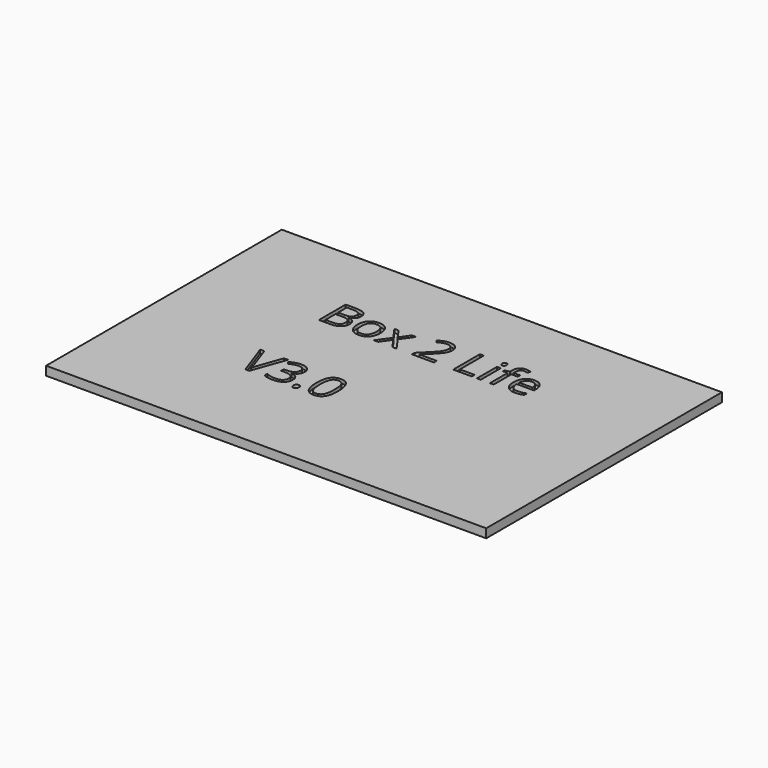
from build123d import *

# Parameters (mm, degrees)
F0_W         = 124
F0_H         = 83
F1_DEPTH     = 2.5
F2_TEXT_SIZE = 13.1944444444
F3_DEPTH     = 1


# Not quite as in the source:
# - Text() gives the source's letters only with a copy of the font that has no kerning and outlines rounded to 1/6400 em; it was checked with that copy


with BuildPart() as f1:
    # F0 (on Top) → F1 (new body)
    with BuildSketch(Plane.XY):
        with Locations((62, 41.5)):
            Rectangle(F0_W, F0_H)
    extrude(amount=F1_DEPTH)

    # F2 (on face) → F3 (cut)
    with BuildSketch(Plane.XY.offset(2.5)):
        with Locations((31.9702690972, 54.5)):
            Text('Box 2 Life', F2_TEXT_SIZE, font='Open Sans', text_align=(TextAlign.LEFT, TextAlign.BOTTOM))
        with Locations((31.9702690972, 26)):
            Text('V3.0', F2_TEXT_SIZE, font='Open Sans', text_align=(TextAlign.LEFT, TextAlign.BOTTOM))
    extrude(amount=-F3_DEPTH, mode=Mode.SUBTRACT)


solid = f1.part
